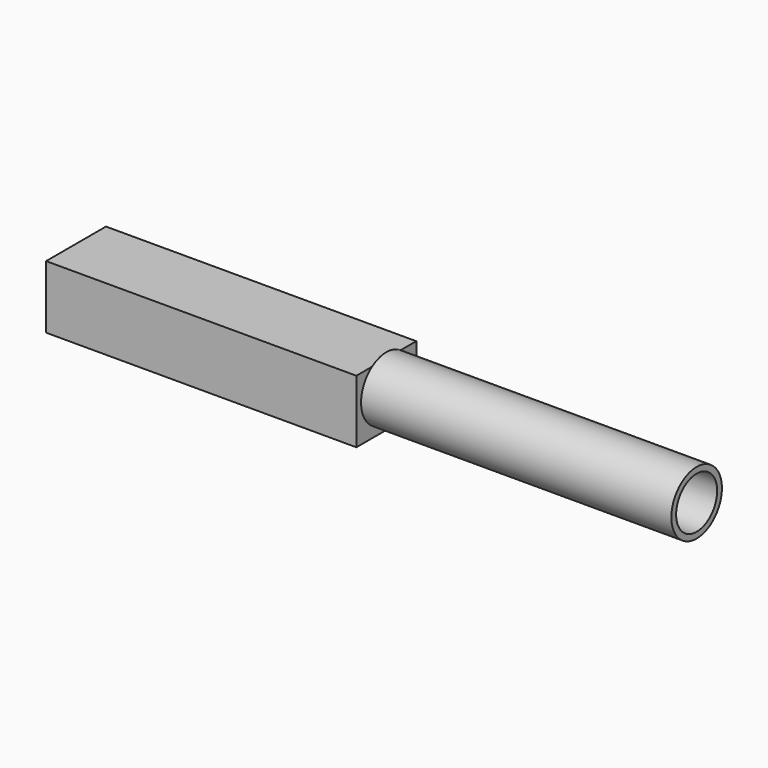
from build123d import *

# Parameters (mm, degrees)
F2_R     = 4.2169292551
F3_DEPTH = 41.402
F4_R     = 3.4205639175
F5_DEPTH = 25.4
F6_W     = 9.9848257378
F6_H     = 8.4082745016
F7_DEPTH = 41.402
F8_W     = 6.5733380616
F8_H     = 5.3974576294
F9_DEPTH = 25.4


# Not quite as in the source:
# - the program builds the solid bodies; features that only make, move or delete a surface that nothing else refers to are left out


with BuildPart() as f3:
    # F2 (on Right) → F3 (new body)
    with BuildSketch(Plane.YZ):
        with Locations((0, -23.187154904)):
            Circle(F2_R)
    extrude(amount=F3_DEPTH)

    # F4 (on face) → F5 (cut)
    with BuildSketch(Plane.YZ.offset(41.402)):
        with Locations((0, -23.187154904)):
            Circle(F4_R)
    extrude(amount=-F5_DEPTH, mode=Mode.SUBTRACT)

    # F6 (on Right) → F7 (join)
    with BuildSketch(Plane.YZ):
        with Locations((0, -23.9110346884)):
            Rectangle(F6_W, F6_H)
    extrude(amount=-F7_DEPTH)

    # F8 (on face) → F9 (cut)
    with BuildSketch(Plane(origin=(-41.402, 0, 0), x_dir=(0, -1, 0), z_dir=(-1, 0, 0))):
        with Locations((0, -23.9110346884)):
            Rectangle(F8_W, F8_H)
    extrude(amount=-F9_DEPTH, mode=Mode.SUBTRACT)


solid = f3.part
